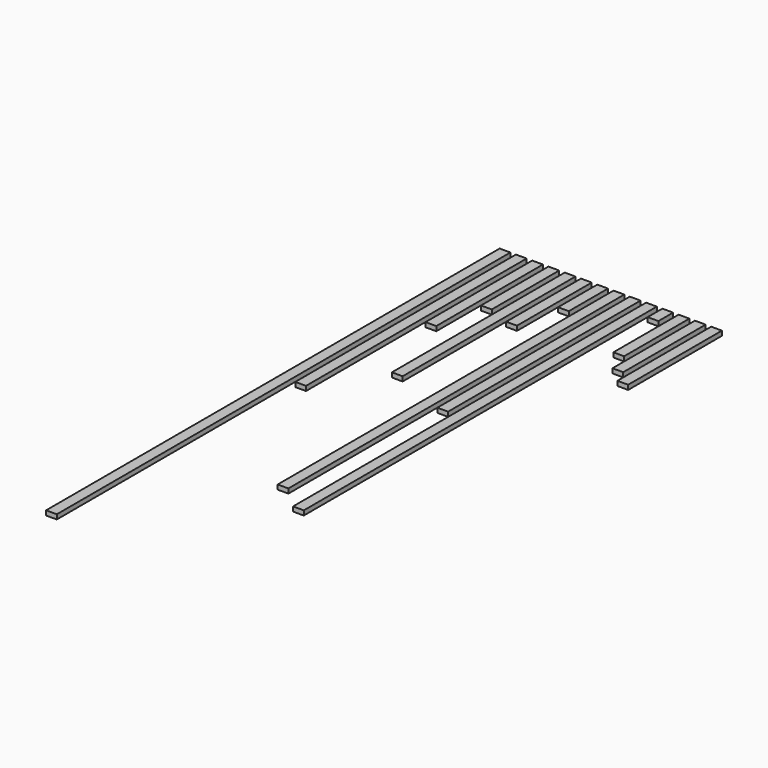
from build123d import *

# Parameters (mm, degrees)
F0_W      = 88.9
F0_H      = 38.1
F2_DEPTH  = 4699
F3_DEPTH  = 2286
F4_DEPTH  = 1104.9
F5_DEPTH  = 698.5
F6_DEPTH  = 1790.7
F7_DEPTH  = 774.7
F8_DEPTH  = 406.4
F9_DEPTH  = 3479.8
F10_DEPTH = 1993.9
F11_DEPTH = 3657.6
F12_DEPTH = 152.4
F13_DEPTH = 676.275
F14_DEPTH = 854.075
F15_DEPTH = 971.55


# Not quite as in the source:
# - a feature of the source that left no trace in its solid (it failed there, or was rolled back) is left out


with BuildPart() as f2:
    # F0 (on Front) → F2 (new body)
    with BuildSketch(Plane.XZ):
        with Locations((134.874, 0)):
            Rectangle(F0_W, F0_H)
    extrude(amount=F2_DEPTH)


with BuildPart() as f3:
    # F0 (on Front) → F3 (new body)
    with BuildSketch(Plane.XZ):
        with Locations((269.748, 0)):
            Rectangle(F0_W, F0_H)
    extrude(amount=F3_DEPTH)


with BuildPart() as f4:
    # F0 (on Front) → F4 (new body)
    with BuildSketch(Plane.XZ):
        with Locations((404.622, 0)):
            Rectangle(F0_W, F0_H)
    extrude(amount=F4_DEPTH)


with BuildPart() as f5:
    # F0 (on Front) → F5 (new body)
    with BuildSketch(Plane.XZ):
        with Locations((539.496, 0)):
            Rectangle(F0_W, F0_H)
    extrude(amount=F5_DEPTH)


with BuildPart() as f6:
    # F0 (on Front) → F6 (new body)
    with BuildSketch(Plane.XZ):
        with Locations((674.37, 0)):
            Rectangle(F0_W, F0_H)
    extrude(amount=F6_DEPTH)


with BuildPart() as f7:
    # F0 (on Front) → F7 (new body)
    with BuildSketch(Plane.XZ):
        with Locations((809.244, 0)):
            Rectangle(F0_W, F0_H)
    extrude(amount=F7_DEPTH)


with BuildPart() as f8:
    # F0 (on Front) → F8 (new body)
    with BuildSketch(Plane.XZ):
        with Locations((944.118, 0)):
            Rectangle(F0_W, F0_H)
    extrude(amount=F8_DEPTH)


with BuildPart() as f9:
    # F0 (on Front) → F9 (new body)
    with BuildSketch(Plane.XZ):
        with Locations((1078.992, 0)):
            Rectangle(F0_W, F0_H)
    extrude(amount=F9_DEPTH)


with BuildPart() as f10:
    # F0 (on Front) → F10 (new body)
    with BuildSketch(Plane.XZ):
        with Locations((1213.866, 0)):
            Rectangle(F0_W, F0_H)
    extrude(amount=F10_DEPTH)


with BuildPart() as f11:
    # F0 (on Front) → F11 (new body)
    with BuildSketch(Plane.XZ):
        with Locations((1348.74, 0)):
            Rectangle(F0_W, F0_H)
    extrude(amount=F11_DEPTH)


with BuildPart() as f12:
    # F0 (on Front) → F12 (new body)
    with BuildSketch(Plane.XZ):
        with Locations((1483.614, 0)):
            Rectangle(F0_W, F0_H)
    extrude(amount=F12_DEPTH)


with BuildPart() as f13:
    # F0 (on Front) → F13 (new body)
    with BuildSketch(Plane.XZ):
        with Locations((1618.488, 0)):
            Rectangle(F0_W, F0_H)
    extrude(amount=F13_DEPTH)


with BuildPart() as f14:
    # F0 (on Front) → F14 (new body)
    with BuildSketch(Plane.XZ):
        with Locations((1753.362, 0)):
            Rectangle(F0_W, F0_H)
    extrude(amount=F14_DEPTH)


with BuildPart() as f15:
    # F0 (on Front) → F15 (new body)
    with BuildSketch(Plane.XZ):
        with Locations((1888.236, 0)):
            Rectangle(F0_W, F0_H)
    extrude(amount=F15_DEPTH)


solid = Compound([f2.part, f3.part, f4.part, f5.part, f6.part, f7.part, f8.part, f9.part, f10.part, f11.part, f12.part, f13.part, f14.part, f15.part])
